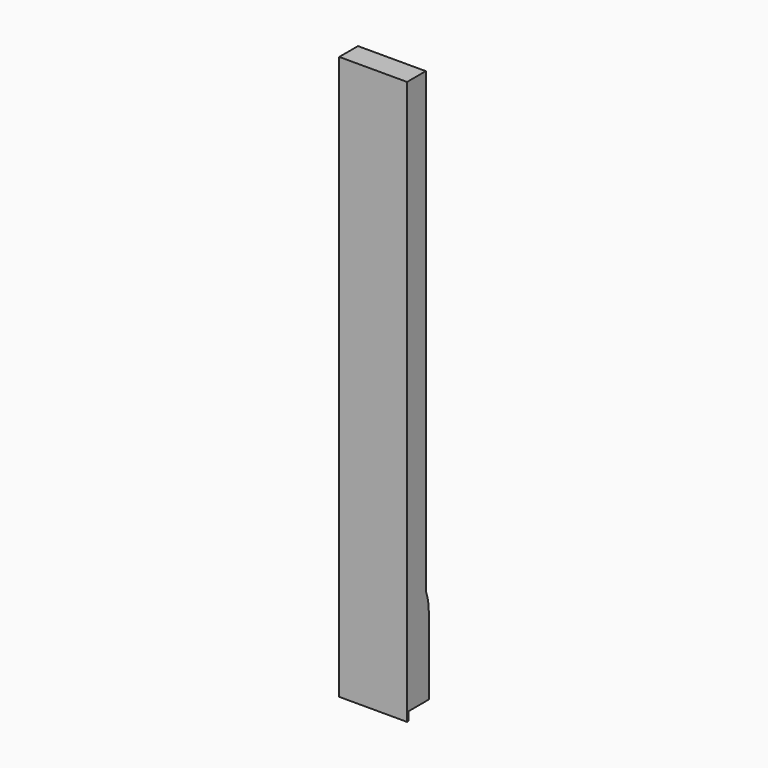
from build123d import *

# Parameters (mm, degrees)
F0_W        = 55
F0_H        = 450
F1_DEPTH    = 22
F2_W        = 55
F2_H        = 1.5
F3_DEPTH    = 7
F4_W        = 3
F4_H        = 375
F5_DEPTH    = 55.001
F6_T1_DEPTH = 55
F7_R        = 40


# Not quite as in the source:
# - a fillet or chamfer that OpenCascade refuses, or shapes differently, is made with other operations: its cross-section is extruded or revolved along the edge and cut away or added


with BuildPart() as f1:
    # F0 (on Front) → F1 (new body)
    with BuildSketch(Plane.XZ):
        Rectangle(F0_W, F0_H)
    extrude(amount=F1_DEPTH)

    # F2 (on face) → F3 (join)
    with BuildSketch(Plane(origin=(0, 0, -225), x_dir=(1, 0, 0), z_dir=(0, 0, -1))):
        with Locations((0, 21.25)):
            Rectangle(F2_W, F2_H)
    extrude(amount=F3_DEPTH)

    # F4 (on face) → F5 (cut, through all)
    with BuildSketch(Plane(origin=(-27.5, 0, 0), x_dir=(0, -1, 0), z_dir=(-1, 0, 0))):
        with Locations((1.5, 37.5)):
            Rectangle(F4_W, F4_H)
    extrude(amount=-F5_DEPTH, mode=Mode.SUBTRACT)

    # F6: fillet of radius 5 on 1 edges, made by hand

    # F6_s2 → F6_t1 (join)
    with BuildSketch(Plane.YZ.offset(-27.5)):
        with BuildLine():
            ThreePointArc((-3, -145.417424305), (-2.1833001327, -148.1560370926), (0, -150))
            Line((0, -150), (-3, -150))
            Line((-3, -150), (-3, -145.417424305))
        make_face()
    extrude(amount=F6_T1_DEPTH)

    # F7
    f7_edges = [f1.edges().sort_by_distance(p)[0] for p in [
        (0, 0, -150),
    ]]
    fillet(f7_edges, radius=F7_R)


solid = f1.part
